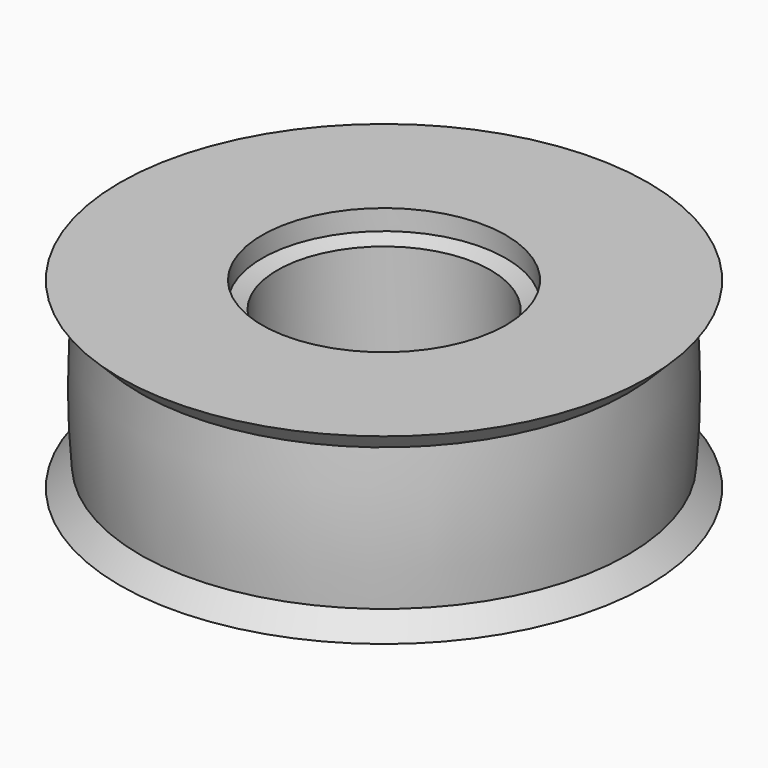
from build123d import *


# Not quite as in the source:
# - a feature names something its author has since deleted; it is built from what else it names


with BuildPart() as f1:
    # F0 (on Front) → F1 (revolve)
    with BuildSketch(Plane.XZ):
        Polygon((6, -9), (13, -9), (12, -8), (12, -1), (13, 0), (6, 0), (6, -1), (5.25, -1.2729776757), (5.25, -7.7270223243), (6, -8), align=None)
        with BuildLine():
            Line((12, -1), (12, -8))
            ThreePointArc((12, -8), (12.1528330258, -4.5), (12, -1))
        make_face()
    revolve(axis=Axis((0, 0, -4.5), (0, 0, -1)))


solid = f1.part
